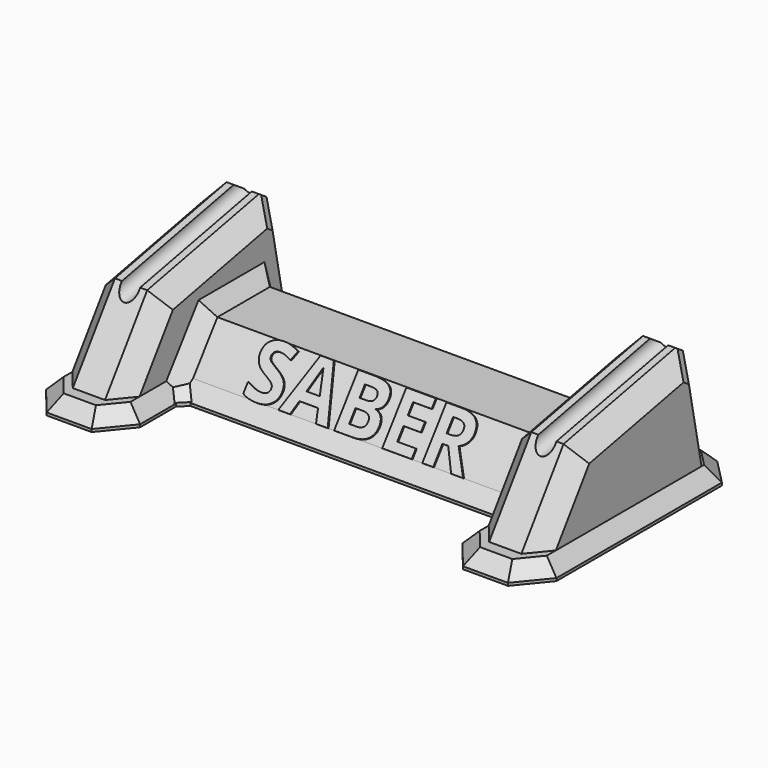
from build123d import *

# Parameters (mm, degrees)
F1_DEPTH       = 12.5
F2_R           = 3.4
F3_DEPTH       = 86.0463297252
F4_SIZE        = 6.5
F5_T1_DEPTH    = 18.0670635836
F5_T3_DEPTH    = 18.0670635836
F5_T5_DEPTH    = 20.4431002518
F5_T7_DEPTH    = 20.4431002518
F7_DEPTH       = 6
F8_SIZE        = 4.99999
F12_DEPTH      = 65
F12_DEPTH_BACK = 65
F13_T4_DEPTH   = 44.9097441071
F13_T10_DEPTH  = 50.1336123214
F13_T16_DEPTH  = 39.2761367259
F13_T21_DEPTH  = 39.2761367259
F13_T26_DEPTH  = 39.2761367259
F13_T31_DEPTH  = 39.2761367259
F13_T36_DEPTH  = 44.9097441071
F13_T42_DEPTH  = 50.1336123214
F13_T48_DEPTH  = 41.8951652993
F13_T54_DEPTH  = 23.9681867216
F13_T59_DEPTH  = 23.9681867216
F13_T64_DEPTH  = 41.8951652993
F13_T70_DEPTH  = 23.9681867216
F13_T75_DEPTH  = 23.9681867216
F13_T81_DEPTH  = 44.9097441071
F13_T86_DEPTH  = 50.1336123214
F13_T93_DEPTH  = 41.8951652993
F13_T97_DEPTH  = 50.1336123214
F13_T105_DEPTH = 44.9097441071
F13_T110_DEPTH = 50.1336123214
F13_T117_DEPTH = 41.8951652993
F13_T121_DEPTH = 50.1336123214
F14_C1_SIZE    = 3
F14_C2_SIZE    = 3
F14_C3_SIZE    = 3
F14_C4_SIZE    = 3
F15_TEXT_SIZE  = 26.6568253159
F16_DEPTH      = 0.5


# Not quite as in the source:
# - a fillet or chamfer that OpenCascade refuses, or shapes differently, is made with other operations: its cross-section is extruded or revolved along the edge and cut away or added
# - a fillet or chamfer is up to 0.001 mm smaller than in the source, because OpenCascade refuses the exact size
# - Text() gives the source's letters only with a copy of the font that has no kerning and outlines rounded to 1/6400 em; it was checked with that copy


with BuildPart() as f1:
    # F0 (on Right) → F1 (new body, symmetric)
    with BuildSketch(Plane.YZ):
        Polygon((-49.9434429395, 0), (37.8115169209, 0), (28.7966039032, 45), (-26.11241175, 34), align=None)
    extrude(amount=F1_DEPTH, both=True)

    # F2 (on face) → F3 (cut, through all)
    with BuildSketch(Plane(origin=(0, 36.352590407, 7.2825653441), x_dir=(-1, 0, 0), z_dir=(0, 0.9805181367, 0.1964285714))):
        with Locations((0, 37.9668403832)):
            Circle(F2_R)
    extrude(amount=-F3_DEPTH, mode=Mode.SUBTRACT)

    # F4
    f4_edges = [f1.edges().sort_by_distance(p)[0] for p in [
        (-12.5, 1.342096, 39.5),
        (-12.5, 33.30406, 22.5),
        (12.5, 33.30406, 22.5),
        (12.5, 1.342096, 39.5),
        (12.5, -38.027927, 17),
        (-12.5, -38.027927, 17),
    ]]
    chamfer(f4_edges, length=F4_SIZE)

    # F5: chamfer of 3 on 4 edges, made by hand

    # F5_s2 → F5_t1 (cut)
    with BuildSketch(Plane.YZ.offset(-4.3520146197)):
        Polygon((25.8550494932, 44.4107142857), (29.3858896175, 42.05844559), (28.7966039032, 45), align=None)
    extrude(amount=F5_T1_DEPTH, mode=Mode.SUBTRACT)

    # F5_s4 → F5_t3 (cut)
    with BuildSketch(Plane.YZ.offset(-13.7150489639)):
        Polygon((25.8550494932, 44.4107142857), (29.3858896175, 42.05844559), (28.7966039032, 45), align=None)
    extrude(amount=F5_T3_DEPTH, mode=Mode.SUBTRACT)

    # F5_s6 → F5_t5 (cut)
    with BuildSketch(Plane(origin=(14.0291581162, 11.000116488, 16.5115714622), x_dir=(-0.617030713, 0.7869390696, 0), z_dir=(0.5773502692, 0.4526943216, 0.6795104987))):
        Polygon((24.7265291494, 24.7159409507), (26.6912649688, 22.4488253472), (26.3633569611, 24.1495535261), align=None)
    extrude(amount=F5_T5_DEPTH, mode=Mode.SUBTRACT)

    # F5_s8 → F5_t7 (cut)
    with BuildSketch(Plane(origin=(-25.8319875497, 20.254591887, 30.4028727101), x_dir=(0.617030713, 0.7869390696, 0), z_dir=(0.5773502692, -0.4526943216, -0.6795104987))):
        Polygon((26.6912649688, 22.4488253472), (24.7265291494, 24.7159409507), (26.3633569611, 24.1495535261), align=None)
    extrude(amount=F5_T7_DEPTH, mode=Mode.SUBTRACT)

    # F6 (on face) → F7 (join)
    with BuildSketch(Plane(origin=(0, 0, 0), x_dir=(1, 0, 0), z_dir=(0, 0, -1))):
        Polygon((-17.5, 43.7917747174), (-17.5, -33.2246846688), (-8.0999371037, -42.8115169209), (8.0999371037, -42.8115169209), (17.5, -33.2246846688), (17.5, 43.7917747174), (8.3681146784, 54.9434429395), (-8.3681146784, 54.9434429395), align=None)
        Polygon((-6, 49.9434429395), (6, 49.9434429395), (12.5, 42.0057782743), (12.5, -31.1823687624), (6, -37.8115169209), (-6, -37.8115169209), (-12.5, -31.1823687624), (-12.5, 42.0057782743), align=None, mode=Mode.SUBTRACT)
        Polygon((12.5, 42.0057782743), (6, 49.9434429395), (-6, 49.9434429395), (-12.5, 42.0057782743), (-12.5, -31.1823687624), (-6, -37.8115169209), (6, -37.8115169209), (12.5, -31.1823687624), align=None)
    extrude(amount=-F7_DEPTH)

    # F8 (size 5 in the source; OpenCascade refuses exactly that, so slightly less here)
    f8_edges = [f1.edges().sort_by_distance(p)[0] for p in [
        (-12.934057, -49.367609, 6),
        (0, -54.943443, 6),
        (-17.5, -5.283545, 6),
        (12.934057, -49.367609, 6),
        (17.5, -5.283545, 6),
        (-12.799969, 38.018101, 6),
        (0, 42.811517, 6),
        (12.799969, 38.018101, 6),
    ]]
    chamfer(f8_edges, length=F8_SIZE)


with BuildPart() as f10_1:
    # F10: instance of F1
    add(f1.part.mirror(Plane.YZ.offset(77.5)))


with BuildPart() as f1_1:
    add(f1.part)

    add(f10_1.part)  # F12 merges F10_1
    # F11 (on offset) → F12 (join, two sides)
    with BuildSketch(Plane.YZ.offset(77.5)) as f12_sk:
        Polygon((-24.1603925824, 1), (-24.1603925824, 0), (26.309485659, 0), (26.309485659, 1), (21.309485659, 6), (16.6040859327, 21.4789453894), (-7.8126965091, 21.4789453894), (-19.1603925824, 6), align=None)
    extrude(amount=F12_DEPTH)
    extrude(f12_sk.sketch, amount=-F12_DEPTH_BACK)

    # F13: chamfer of 5 on 10 edges, made by hand


with BuildPart() as f13_tool2:
    # F13_s3 → F13_t4 (new body)
    with BuildSketch(Plane(origin=(0, 15.1132721955, 20.6154195051), x_dir=(1, 0, 0), z_dir=(0, -0.5912440362, -0.806492709))):
        Polygon((17.5, 19.0001811367), (12.5, 24.0001811367), (12.5, 19.0001811367), align=None)
    extrude(amount=F13_T4_DEPTH)

    split(bisect_by=Plane.XY.offset(21.4789453894), keep=Keep.BOTTOM)

    split(bisect_by=Plane.XY, keep=Keep.TOP)


with BuildPart() as f1_2:
    add(f1_1.part)

    # F13_t1: union F13_tool2
    add(f13_tool2.part)


with BuildPart() as f13_tool8:
    # F13_s9 → F13_t10 (new body)
    with BuildSketch(Plane.XZ.offset(-29.4625008725)):
        Polygon((12.5, 26.4789453894), (17.5, 21.4789453894), (12.5, 21.4789453894), align=None)
    extrude(amount=F13_T10_DEPTH)

    split(bisect_by=Plane(origin=(0, -15.323507557, 11.2337437829), x_dir=(1, 0, 0), z_dir=(0, 0.806492709, -0.5912440362)), keep=Keep.TOP)

    split(bisect_by=Plane(origin=(0, 21.176524643, 6.4373903229), x_dir=(1, 0, 0), z_dir=(0, -0.9567699635, -0.290845727)), keep=Keep.TOP)


with BuildPart() as f1_3:
    add(f1_2.part)

    # F13_t7: union F13_tool8
    add(f13_tool8.part)


with BuildPart() as f13_tool14:
    # F13_s15 → F13_t16 (new body)
    with BuildSketch(Plane(origin=(17.9724820553, -17.9724820553, -17.9724820553), x_dir=(-0.7071067812, -0.7071067812, 0), z_dir=(-0.5773502692, 0.5773502692, 0.5773502692))):
        Polygon((2.2096016893, 19.2676603882), (7.2096016893, 19.2676603882), (4.7096016893, 17.8242847152), align=None)
    extrude(amount=F13_T16_DEPTH)

    split(bisect_by=Plane.YZ.offset(17.5), keep=Keep.BOTTOM)


with BuildPart() as f1_4:
    add(f1_3.part)

    # F13_t13: union F13_tool14
    add(f13_tool14.part)


with BuildPart() as f13_tool19:
    # F13_s20 → F13_t21 (new body)
    with BuildSketch(Plane(origin=(17.9724820553, -17.9724820553, -17.9724820553), x_dir=(-0.7071067812, -0.7071067812, 0), z_dir=(-0.5773502692, 0.5773502692, 0.5773502692))):
        Polygon((2.2096016893, 19.2676603882), (7.2096016893, 19.2676603882), (4.7096016893, 17.8242847152), align=None)
    extrude(amount=F13_T21_DEPTH)

    split(bisect_by=Plane.XZ.offset(24.1603925824), keep=Keep.BOTTOM)


with BuildPart() as f1_5:
    add(f1_4.part)

    # F13_t18: union F13_tool19
    add(f13_tool19.part)


with BuildPart() as f13_tool24:
    # F13_s25 → F13_t26 (new body)
    with BuildSketch(Plane(origin=(33.6941846113, 33.6941846113, 33.6941846113), x_dir=(-0.7071067812, 0.7071067812, 0), z_dir=(0.5773502692, 0.5773502692, 0.5773502692))):
        Polygon((-116.8111527732, -44.0108246337), (-111.8111527732, -44.0108246337), (-114.3111527732, -45.4542003067), align=None)
    extrude(amount=F13_T26_DEPTH)

    split(bisect_by=Plane.XZ.offset(24.1603925824), keep=Keep.BOTTOM)


with BuildPart() as f1_6:
    add(f1_5.part)

    # F13_t23: union F13_tool24
    add(f13_tool24.part)


with BuildPart() as f13_tool29:
    # F13_s30 → F13_t31 (new body)
    with BuildSketch(Plane(origin=(33.6941846113, 33.6941846113, 33.6941846113), x_dir=(-0.7071067812, 0.7071067812, 0), z_dir=(0.5773502692, 0.5773502692, 0.5773502692))):
        Polygon((-116.8111527732, -44.0108246337), (-111.8111527732, -44.0108246337), (-114.3111527732, -45.4542003067), align=None)
    extrude(amount=F13_T31_DEPTH)

    split(bisect_by=Plane.YZ.offset(137.5), keep=Keep.TOP)


with BuildPart() as f1_7:
    add(f1_6.part)

    # F13_t28: union F13_tool29
    add(f13_tool29.part)


with BuildPart() as f13_tool34:
    # F13_s35 → F13_t36 (new body)
    with BuildSketch(Plane(origin=(0, 15.1132721955, 20.6154195051), x_dir=(1, 0, 0), z_dir=(0, -0.5912440362, -0.806492709))):
        Polygon((137.5, 19.0001811367), (142.5, 24.0001811367), (142.5, 19.0001811367), align=None)
    extrude(amount=F13_T36_DEPTH)

    split(bisect_by=Plane.XY.offset(21.4789453894), keep=Keep.BOTTOM)

    split(bisect_by=Plane.XY, keep=Keep.TOP)


with BuildPart() as f1_8:
    add(f1_7.part)

    # F13_t33: union F13_tool34
    add(f13_tool34.part)


with BuildPart() as f13_tool40:
    # F13_s41 → F13_t42 (new body)
    with BuildSketch(Plane.XZ.offset(-29.4625008725)):
        Polygon((142.5, 26.4789453894), (137.5, 21.4789453894), (142.5, 21.4789453894), align=None)
    extrude(amount=F13_T42_DEPTH)

    split(bisect_by=Plane(origin=(0, -15.323507557, 11.2337437829), x_dir=(1, 0, 0), z_dir=(0, 0.806492709, -0.5912440362)), keep=Keep.TOP)

    split(bisect_by=Plane(origin=(0, 21.176524643, 6.4373903229), x_dir=(1, 0, 0), z_dir=(0, -0.9567699635, -0.290845727)), keep=Keep.TOP)


with BuildPart() as f1_9:
    add(f1_8.part)

    # F13_t39: union F13_tool40
    add(f13_tool40.part)


with BuildPart() as f13_tool46:
    # F13_s47 → F13_t48 (new body)
    with BuildSketch(Plane(origin=(0, 3.8727760569, -12.7399355159), x_dir=(1, 0, 0), z_dir=(0, -0.290845727, 0.9567699635))):
        Polygon((142.5, 27.1333501785), (137.5, 22.1333501785), (142.5, 22.1333501785), align=None)
    extrude(amount=F13_T48_DEPTH)

    split(bisect_by=Plane.XY.offset(21.4789453894), keep=Keep.BOTTOM)

    split(bisect_by=Plane.XY, keep=Keep.TOP)


with BuildPart() as f1_10:
    add(f1_9.part)

    # F13_t45: union F13_tool46
    add(f13_tool46.part)


with BuildPart() as f13_tool52:
    # F13_s53 → F13_t54 (new body)
    with BuildSketch(Plane(origin=(46.8158593082, -46.8158593082, 46.8158593082), x_dir=(-0.7071067812, -0.7071067812, 0), z_dir=(-0.5773502692, 0.5773502692, -0.5773502692))):
        Polygon((-118.3307910611, -43.1334610591), (-113.3307910611, -43.1334610591), (-115.8307910611, -44.5768367321), align=None)
    extrude(amount=F13_T54_DEPTH)

    split(bisect_by=Plane.XZ.offset(-26.309485659), keep=Keep.TOP)


with BuildPart() as f1_11:
    add(f1_10.part)

    # F13_t51: union F13_tool52
    add(f13_tool52.part)


with BuildPart() as f13_tool57:
    # F13_s58 → F13_t59 (new body)
    with BuildSketch(Plane(origin=(46.8158593082, -46.8158593082, 46.8158593082), x_dir=(-0.7071067812, -0.7071067812, 0), z_dir=(-0.5773502692, 0.5773502692, -0.5773502692))):
        Polygon((-118.3307910611, -43.1334610591), (-113.3307910611, -43.1334610591), (-115.8307910611, -44.5768367321), align=None)
    extrude(amount=F13_T59_DEPTH)

    split(bisect_by=Plane.YZ.offset(137.5), keep=Keep.TOP)


with BuildPart() as f1_12:
    add(f1_11.part)

    # F13_t56: union F13_tool57
    add(f13_tool57.part)


with BuildPart() as f13_tool62:
    # F13_s63 → F13_t64 (new body)
    with BuildSketch(Plane(origin=(0, 3.8727760569, -12.7399355159), x_dir=(1, 0, 0), z_dir=(0, -0.290845727, 0.9567699635))):
        Polygon((17.5, 22.1333501785), (12.5, 27.1333501785), (12.5, 22.1333501785), align=None)
    extrude(amount=F13_T64_DEPTH)

    split(bisect_by=Plane.XY.offset(21.4789453894), keep=Keep.BOTTOM)

    split(bisect_by=Plane.XY, keep=Keep.TOP)


with BuildPart() as f1_13:
    add(f1_12.part)

    # F13_t61: union F13_tool62
    add(f13_tool62.part)


with BuildPart() as f13_tool68:
    # F13_s69 → F13_t70 (new body)
    with BuildSketch(Plane(origin=(4.8508073585, 4.8508073585, -4.8508073585), x_dir=(-0.7071067812, 0.7071067812, 0), z_dir=(0.5773502692, 0.5773502692, -0.5773502692))):
        Polygon((3.7292399772, 20.1450239628), (8.7292399772, 20.1450239628), (6.2292399772, 18.7016482898), align=None)
    extrude(amount=F13_T70_DEPTH)

    split(bisect_by=Plane.YZ.offset(17.5), keep=Keep.BOTTOM)


with BuildPart() as f1_14:
    add(f1_13.part)

    # F13_t67: union F13_tool68
    add(f13_tool68.part)


with BuildPart() as f13_tool73:
    # F13_s74 → F13_t75 (new body)
    with BuildSketch(Plane(origin=(4.8508073585, 4.8508073585, -4.8508073585), x_dir=(-0.7071067812, 0.7071067812, 0), z_dir=(0.5773502692, 0.5773502692, -0.5773502692))):
        Polygon((3.7292399772, 20.1450239628), (8.7292399772, 20.1450239628), (6.2292399772, 18.7016482898), align=None)
    extrude(amount=F13_T75_DEPTH)

    split(bisect_by=Plane.XZ.offset(-26.309485659), keep=Keep.TOP)


with BuildPart() as f1_15:
    add(f1_14.part)

    # F13_t72: union F13_tool73
    add(f13_tool73.part)


with BuildPart() as f13_tool79:
    # F13_s80 → F13_t81 (new body)
    with BuildSketch(Plane(origin=(0, 15.1132721955, 20.6154195051), x_dir=(1, 0, 0), z_dir=(0, -0.5912440362, -0.806492709))):
        Polygon((17.5, 19.0001811367), (12.5, 24.0001811367), (12.5, 19.0001811367), align=None)
    extrude(amount=F13_T81_DEPTH)

    split(bisect_by=Plane.XY.offset(21.4789453894), keep=Keep.TOP)

    split(bisect_by=Plane(origin=(22.2334201916, -4.3672789662, 21.8002717379), x_dir=(-0.192745304, -0.9812488205, 0), z_dir=(-0.7071067812, 0.1388959749, -0.6933310235)), keep=Keep.TOP)


with BuildPart() as f13_tool84:
    # F13_s85 → F13_t86 (new body)
    with BuildSketch(Plane.XZ.offset(-29.4625008725)):
        Polygon((12.5, 26.4789453894), (17.5, 21.4789453894), (12.5, 21.4789453894), align=None)
    extrude(amount=F13_T86_DEPTH)

    split(bisect_by=Plane(origin=(0, -15.323507557, 11.2337437829), x_dir=(1, 0, 0), z_dir=(0, -0.806492709, 0.5912440362)), keep=Keep.TOP)


with BuildPart() as f13_tool79_1:
    add(f13_tool79.part)

    # F13_t88: intersect F13_tool84
    add(f13_tool84.part, mode=Mode.INTERSECT)


with BuildPart() as f1_16:
    add(f1_15.part)

    # F13_t77: union F13_tool79
    add(f13_tool79_1.part)


with BuildPart() as f13_tool91:
    # F13_s92 → F13_t93 (new body)
    with BuildSketch(Plane(origin=(0, 3.8727760569, -12.7399355159), x_dir=(1, 0, 0), z_dir=(0, -0.290845727, 0.9567699635))):
        Polygon((17.5, 22.1333501785), (12.5, 27.1333501785), (12.5, 22.1333501785), align=None)
    extrude(amount=F13_T93_DEPTH)

    split(bisect_by=Plane.XY.offset(21.4789453894), keep=Keep.TOP)


with BuildPart() as f13_tool95:
    # F13_s96 → F13_t97 (new body)
    with BuildSketch(Plane.XZ.offset(-29.4625008725)):
        Polygon((12.5, 26.4789453894), (17.5, 21.4789453894), (12.5, 21.4789453894), align=None)
    extrude(amount=F13_T97_DEPTH)

    split(bisect_by=Plane(origin=(0, 21.176524643, 6.4373903229), x_dir=(1, 0, 0), z_dir=(0, 0.9567699635, 0.290845727)), keep=Keep.TOP)

    split(bisect_by=Plane(origin=(21.5374390578, 21.1178496135, 4.2305683864), x_dir=(0.7001172766, -0.7140278699, 0), z_dir=(-0.7071067812, -0.6933310235, -0.1388959749)), keep=Keep.TOP)


with BuildPart() as f13_tool91_1:
    add(f13_tool91.part)

    # F13_t100: intersect F13_tool95
    add(f13_tool95.part, mode=Mode.INTERSECT)


with BuildPart() as f1_17:
    add(f1_16.part)

    # F13_t89: union F13_tool91
    add(f13_tool91_1.part)


with BuildPart() as f13_tool103:
    # F13_s104 → F13_t105 (new body)
    with BuildSketch(Plane(origin=(0, 15.1132721955, 20.6154195051), x_dir=(1, 0, 0), z_dir=(0, -0.5912440362, -0.806492709))):
        Polygon((137.5, 19.0001811367), (142.5, 24.0001811367), (142.5, 19.0001811367), align=None)
    extrude(amount=F13_T105_DEPTH)

    split(bisect_by=Plane.XY.offset(21.4789453894), keep=Keep.TOP)

    split(bisect_by=Plane(origin=(55.2665798084, 10.8559353195, -54.1898838535), x_dir=(-0.192745304, 0.9812488205, 0), z_dir=(0.7071067812, 0.1388959749, -0.6933310235)), keep=Keep.TOP)


with BuildPart() as f13_tool108:
    # F13_s109 → F13_t110 (new body)
    with BuildSketch(Plane.XZ.offset(-29.4625008725)):
        Polygon((142.5, 26.4789453894), (137.5, 21.4789453894), (142.5, 21.4789453894), align=None)
    extrude(amount=F13_T110_DEPTH)

    split(bisect_by=Plane(origin=(0, -15.323507557, 11.2337437829), x_dir=(1, 0, 0), z_dir=(0, -0.806492709, 0.5912440362)), keep=Keep.TOP)


with BuildPart() as f13_tool103_1:
    add(f13_tool103.part)

    # F13_t112: intersect F13_tool108
    add(f13_tool108.part, mode=Mode.INTERSECT)


with BuildPart() as f1_18:
    add(f1_17.part)

    # F13_t101: union F13_tool103
    add(f13_tool103_1.part)


with BuildPart() as f13_tool115:
    # F13_s116 → F13_t117 (new body)
    with BuildSketch(Plane(origin=(0, 3.8727760569, -12.7399355159), x_dir=(1, 0, 0), z_dir=(0, -0.290845727, 0.9567699635))):
        Polygon((142.5, 27.1333501785), (137.5, 22.1333501785), (142.5, 22.1333501785), align=None)
    extrude(amount=F13_T117_DEPTH)

    split(bisect_by=Plane.XY.offset(21.4789453894), keep=Keep.TOP)


with BuildPart() as f13_tool119:
    # F13_s120 → F13_t121 (new body)
    with BuildSketch(Plane.XZ.offset(-29.4625008725)):
        Polygon((142.5, 26.4789453894), (137.5, 21.4789453894), (142.5, 21.4789453894), align=None)
    extrude(amount=F13_T121_DEPTH)

    split(bisect_by=Plane(origin=(55.9625609422, -54.8723059779, -10.9926458994), x_dir=(0.7001172766, 0.7140278699, 0), z_dir=(0.7071067812, -0.6933310235, -0.1388959749)), keep=Keep.TOP)

    split(bisect_by=Plane(origin=(0, 21.176524643, 6.4373903229), x_dir=(1, 0, 0), z_dir=(0, 0.9567699635, 0.290845727)), keep=Keep.TOP)


with BuildPart() as f13_tool115_1:
    add(f13_tool115.part)

    # F13_t124: intersect F13_tool119
    add(f13_tool119.part, mode=Mode.INTERSECT)


with BuildPart() as f1_19:
    add(f1_18.part)

    # F13_t113: union F13_tool115
    add(f13_tool115_1.part)

    # F14: chamfer of 3 on 24 edges, made by hand

    # F14_c1
    f14_c1_edges = [f1_19.edges().sort_by_distance(p)[0] for p in [
        (137.5, 26.309485659, 0.5),
    ]]
    chamfer(f14_c1_edges, length=F14_C1_SIZE)

    # F14_c2
    f14_c2_edges = [f1_19.edges().sort_by_distance(p)[0] for p in [
        (17.5, 26.309485659, 0.5),
    ]]
    chamfer(f14_c2_edges, length=F14_C2_SIZE)

    # F14_c3
    f14_c3_edges = [f1_19.edges().sort_by_distance(p)[0] for p in [
        (17.5, -24.1603925824, 0.5),
    ]]
    chamfer(f14_c3_edges, length=F14_C3_SIZE)

    # F14_c4
    f14_c4_edges = [f1_19.edges().sort_by_distance(p)[0] for p in [
        (137.5, -24.1603925824, 0.5),
    ]]
    chamfer(f14_c4_edges, length=F14_C4_SIZE)

    # F15 (on face) → F16 (join)
    with BuildSketch(Plane(origin=(0, -15.323507557, 11.2337437829), x_dir=(1, 0, 0), z_dir=(0, -0.806492709, 0.5912440362))):
        with Locations((34.8803179621, -6.4895115905)):
            Text('SABER', F15_TEXT_SIZE, font='Open Sans', font_style=FontStyle.BOLD, text_align=(TextAlign.LEFT, TextAlign.BOTTOM))
    extrude(amount=F16_DEPTH)


solid = f1_19.part
